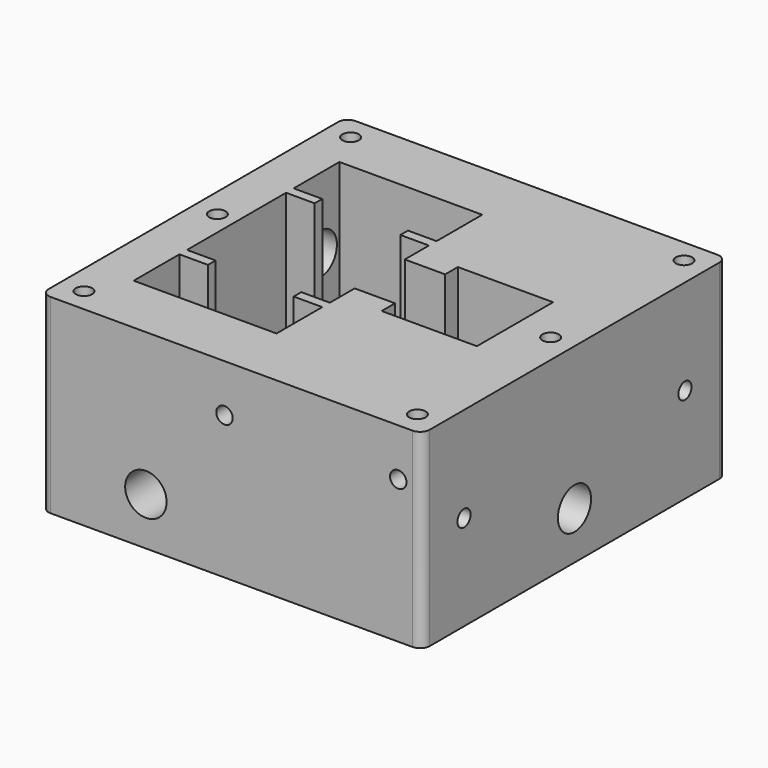
from build123d import *

# Parameters (mm, degrees)
F1_DEPTH  = 40
F2_W      = 20
F2_H      = 20
F3_DEPTH  = 35
F4_R      = 4.35
F5_DEPTH  = 15
F6_R      = 4.35
F7_DEPTH  = 15
F8_W      = 8.4756634911
F8_H      = 13.160008005
F9_DEPTH  = 15
F10_R     = 1.725
F11_DEPTH = 15
F12_R     = 11.5
F13_DEPTH = 2.5
F14_R     = 1.725
F15_DEPTH = 10
F16_R     = 1.725
F17_DEPTH = 10
F18_R     = 1.725
F19_DEPTH = 25
F20_R     = 4.35
F21_DEPTH = 15
F22_R     = 4.35
F23_DEPTH = 15
F24_W     = 18
F24_H     = 2
F25_DEPTH = 6


# Not quite as in the source:
# - a feature names something its author has since deleted; it is built from what else it names


with BuildPart() as f1:
    # F0 (on Top) → F1 (new body)
    with BuildSketch(Plane.XY):
        with BuildLine():
            ThreePointArc((40, 38), (39.4142135624, 39.4142135624), (38, 40))
            Line((38, 40), (-38, 40))
            ThreePointArc((-38, 40), (-39.4142135624, 39.4142135624), (-40, 38))
            Line((-40, 38), (-40, -38))
            ThreePointArc((-40, -38), (-39.4142135624, -39.4142135624), (-38, -40))
            Line((-38, -40), (38, -40))
            ThreePointArc((38, -40), (39.4142135624, -39.4142135624), (40, -38))
            Line((40, -38), (40, 38))
        make_face()
    extrude(amount=F1_DEPTH)

    # F2 (on face) → F3 (cut)
    with BuildSketch(Plane.XY.offset(40)):
        with Locations((17.50956662, 0)):
            Rectangle(F2_W, F2_H)
        Polygon((-24.9660968933, -15), (-30.9660968933, -15), (-30.9660968933, -26.9999999998), (-0.9660968933, -26.9999999998), (-0.9660968933, -15), (-6.9660968933, -15), (-6.9660968933, -13), (-0.9660968933, -13), (-0.9660968933, 13), (-6.9660968933, 13), (-6.9660968933, 15), (-0.9660968933, 15), (-0.9660968933, 26.9999999998), (-30.9660968933, 26.9999999998), (-30.9660968933, 15), (-24.9660968933, 15), (-24.9660968933, 13), (-30.9660968933, 13), (-30.9660968933, -13), (-24.9660968933, -13), align=None)
    extrude(amount=-F3_DEPTH, mode=Mode.SUBTRACT)

    # F4 (on face) → F5 (cut)
    with BuildSketch(Plane(origin=(-40, 0, 0), x_dir=(0, -1, 0), z_dir=(-1, 0, 0))):
        with Locations((-22, 25)):
            Circle(F4_R)
        with Locations((22, 25)):
            Circle(F4_R)
        with Locations((0, 10)):
            Circle(F4_R)
    extrude(amount=-F5_DEPTH, mode=Mode.SUBTRACT)

    # F6 (on face) → F7 (cut)
    with BuildSketch(Plane.YZ.offset(40)):
        with Locations((0, 10)):
            Circle(F6_R)
    extrude(amount=-F7_DEPTH, mode=Mode.SUBTRACT)

    # F8 (on face) → F9 (cut)
    with BuildSketch(Plane.XY.offset(40)):
        with Locations((3.2717348745, 0.0860663135)):
            Rectangle(F8_W, F8_H)
    extrude(amount=-F9_DEPTH, mode=Mode.SUBTRACT)

    # F10 (on face) → F11 (cut)
    with BuildSketch(Plane.XY.offset(40)):
        with Locations((-35, 0)):
            Circle(F10_R)
        with Locations((35, 0)):
            Circle(F10_R)
        with Locations((-35, 35)):
            Circle(F10_R)
        with Locations((-35, -35)):
            Circle(F10_R)
        with Locations((35, 35)):
            Circle(F10_R)
        with Locations((35, -35)):
            Circle(F10_R)
    extrude(amount=-F11_DEPTH, mode=Mode.SUBTRACT)

    # F12 (on face) → F13 (cut)
    with BuildSketch(Plane.XY.offset(5)):
        with Locations((-15.966096893, 0)):
            Circle(F12_R)
    extrude(amount=-F13_DEPTH, mode=Mode.SUBTRACT)

    # F14 (on face) → F15 (cut)
    with BuildSketch(Plane.XZ.offset(40)):
        with Locations((-1.5, 30)):
            Circle(F14_R)
        with Locations((35, 30)):
            Circle(F14_R)
    extrude(amount=-F15_DEPTH, mode=Mode.SUBTRACT)

    # F16 (on face) → F17 (cut)
    with BuildSketch(Plane(origin=(0, 40, 0), x_dir=(-1, 0, 0), z_dir=(0, 1, 0))):
        with Locations((-35, 30)):
            Circle(F16_R)
        with Locations((1.5, 30)):
            Circle(F16_R)
    extrude(amount=-F17_DEPTH, mode=Mode.SUBTRACT)

    # F18 (on face) → F19 (cut)
    with BuildSketch(Plane.YZ.offset(40)):
        with Locations((-29, 20)):
            Circle(F18_R)
        with Locations((29, 20)):
            Circle(F18_R)
    extrude(amount=-F19_DEPTH, mode=Mode.SUBTRACT)

    # F20 (on face) → F21 (cut)
    with BuildSketch(Plane(origin=(0, 40, 0), x_dir=(-1, 0, 0), z_dir=(0, 1, 0))):
        with Locations((18, 10)):
            Circle(F20_R)
    extrude(amount=-F21_DEPTH, mode=Mode.SUBTRACT)

    # F22 (on face) → F23 (cut)
    with BuildSketch(Plane.XZ.offset(40)):
        with Locations((-18, 10)):
            Circle(F22_R)
    extrude(amount=-F23_DEPTH, mode=Mode.SUBTRACT)

    # F24 (on face) → F25 (join)
    with BuildSketch(Plane.XY.offset(5)):
        with Locations((-15.9660968933, 14)):
            Rectangle(F24_W, F24_H)
        with Locations((-15.9660968933, -14)):
            Rectangle(F24_W, F24_H)
    extrude(amount=F25_DEPTH)


solid = f1.part
